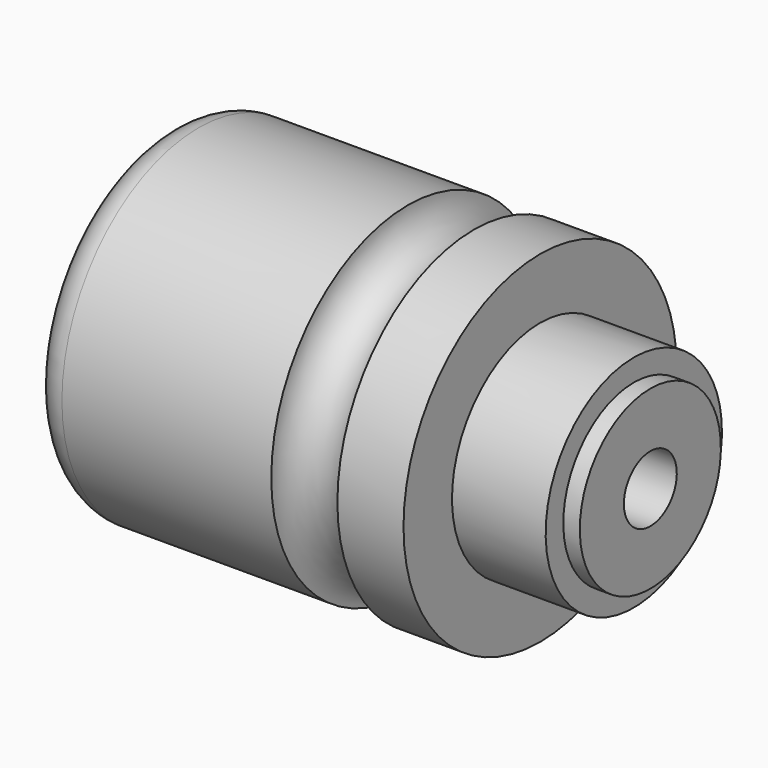
from build123d import *

# Parameters (mm, degrees)
F4_R = 5.99999


# Not quite as in the source:
# - a fillet or chamfer is up to 0.001 mm smaller than in the source, because OpenCascade refuses the exact size


with BuildPart() as f1:
    # F0 (on Front) → F1 (revolve)
    with BuildSketch(Plane.XZ):
        with BuildLine():
            Line((0, 31), (0, 0))
            Line((0, 0), (88, 0))
            Line((88, 0), (88, 16))
            Line((88, 16), (85, 16))
            Line((85, 16), (85, 20))
            Line((85, 20), (68, 20))
            Line((68, 20), (68, 31))
            Line((68, 31), (56, 31))
            ThreePointArc((56, 31), (50, 25), (44, 31))
            Line((44, 31), (0, 31))
        make_face()
    revolve(axis=Axis((-6.5542864613, 0, 0), (-1, 0, 0)))

    # F2 (on Front) → F3 (revolve, cut)
    with BuildSketch(Plane.XZ):
        Polygon((0, 25), (0, 0), (88, 0), (88, 6), (30, 6), (30, 12.5), (22, 12.5), (22, 20.5), (15, 20.5), (15, 12.5), (12, 12.5), (12, 16), (1.5, 16), (1.5, 25), align=None)
    revolve(axis=Axis((44, 0, 0), (-1, 0, 0)), mode=Mode.SUBTRACT)

    # F4 (radius 6 in the source; OpenCascade refuses exactly that, so slightly less here)
    f4_edges = [f1.edges().sort_by_distance(p)[0] for p in [
        (0, 0, -31),
    ]]
    fillet(f4_edges, radius=F4_R)


solid = f1.part
